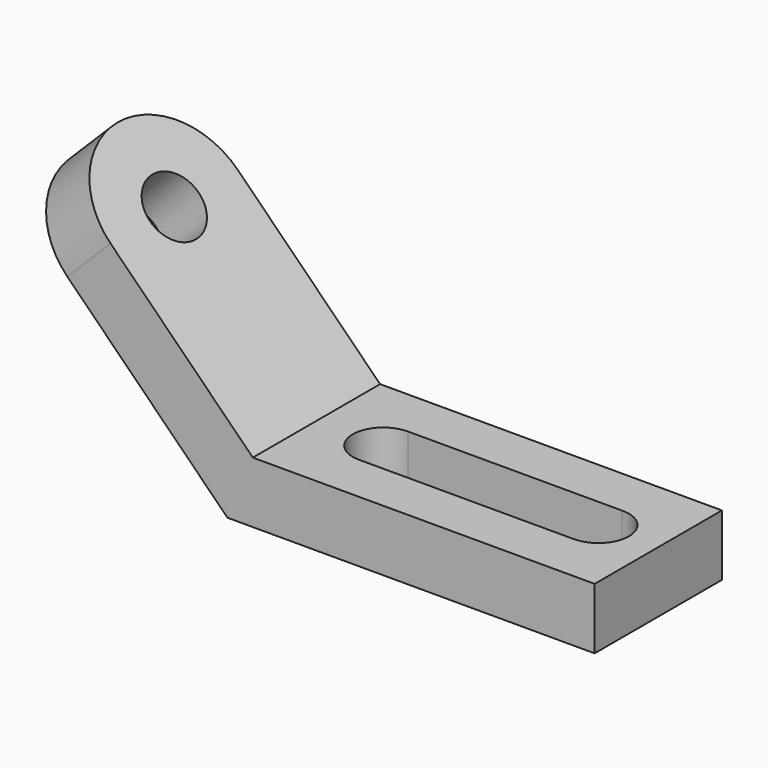
from build123d import *

# Parameters (mm, degrees)
F0_W     = 90
F0_H     = 20
F0_W_2   = 10
F1_DEPTH = 52
F3_D     = 20
F5_D     = 20
F6_R     = 25.99999
F7_DEPTH = 312


# Not quite as in the source:
# - a fillet or chamfer is up to 0.001 mm smaller than in the source, because OpenCascade refuses the exact size


with BuildPart() as f1:
    # F0 (on Front) → F1 (new body)
    with BuildSketch(Plane.XZ):
        Polygon((-16.9582804857, -1.5154299321), (-16.9582804857, 18.4845700679), (-28.6740092382, 18.4845700679), (-68.0709788579, 57.8815396876), (-82.2131144816, 72.0236753113), (-93.5268229806, 83.3373838103), (-107.6689586043, 69.1952481866), (-36.9582804857, -1.5154299321), align=None)
        with Locations((28.0417195143, 8.4845700679)):
            Rectangle(F0_W, F0_H)
        with Locations((78.0417195143, 8.4845700679)):
            Rectangle(F0_W_2, F0_H)
    extrude(amount=F1_DEPTH)

    # F3 (through all)
    with Locations(Plane.XY.offset(18.4845700679)):
        with Locations((63.4629929066, -26), (-6.8132670224, -26)):
            Hole(F3_D / 2)

    # F5 (through all)
    with Locations(Plane(origin=(-5.0947195851, 0, -5.0947195851), x_dir=(0, 1, 0), z_dir=(0.7071067812, 0, 0.7071067812))):
        with Locations((-26, 99.061879971)):
            Hole(F5_D / 2)

    # F6 (radius 26 in the source; OpenCascade refuses exactly that, so slightly less here)
    f6_edges = [f1.edges().sort_by_distance(p)[0] for p in [
        (-100.597891, 0, 76.266316),
        (-100.597891, -52, 76.266316),
    ]]
    fillet(f6_edges, radius=F6_R)

    # F2 (on face) → F7 (cut)
    with BuildSketch(Plane.XY.offset(18.4845700679)):
        Polygon((63.1867329776, -36), (63.1867329776, -26), (52.6720061898, -26), (0, -26), (-5.5663499609, -26), (-6.8132670224, -26), (-6.8132670224, -36), align=None)
        Polygon((52.6720061898, -26), (63.1867329776, -26), (63.1867329776, -16), (-6.8132670224, -16), (-6.8132670224, -26), (-5.5663499609, -26), (0, -26), align=None)
    extrude(amount=-F7_DEPTH, mode=Mode.SUBTRACT)


solid = f1.part
